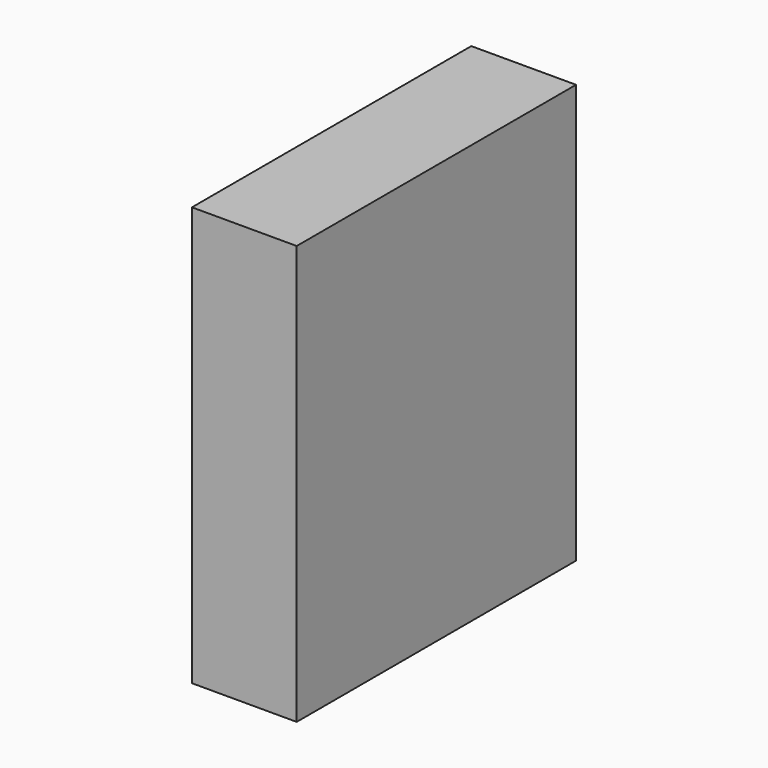
from build123d import *

# Parameters (mm, degrees)
F0_W         = 300
F0_H         = 1000
F1_DEPTH     = 1200
F2_T         = -25
F3_W         = 50
F3_H         = 1150
F4_DEPTH     = 275
F5_TEXT_SIZE = 40.509013666
F6_DEPTH     = 10


# Not quite as in the source:
# - a feature names something its author has since deleted; it is built from what else it names
# - Text() gives the source's letters only with a copy of the font that has no kerning and outlines rounded to 1/6400 em; it was checked with that copy


with BuildPart() as f1:
    # F0 (on Top) → F1 (new body)
    with BuildSketch(Plane.XY):
        Rectangle(F0_W, F0_H)
    extrude(amount=F1_DEPTH)

    # F2
    f2_openings = [f1.faces().sort_by_distance(p)[0] for p in [
        (-150, 0, 600),
    ]]
    offset(amount=F2_T, openings=f2_openings)

    # F3 (on face) → F4 (join)
    with BuildSketch(Plane(origin=(125, 0, 0), x_dir=(0, -1, 0), z_dir=(-1, 0, 0))):
        with Locations((190.852278471, 600)):
            Rectangle(F3_W, F3_H)
        with Locations((-180.2186727524, 600)):
            Rectangle(F3_W, F3_H)
    extrude(amount=F4_DEPTH)

    # F5 (on face) → F6 (join)
    with BuildSketch(Plane(origin=(0, 0, 0), x_dir=(1, 0, 0), z_dir=(0, 0, -1))):
        with Locations((-90.1935100555, 359.3434989452)):
            Text("David's", F5_TEXT_SIZE, font='Open Sans', text_align=(TextAlign.LEFT, TextAlign.BOTTOM))
        with Locations((-90.1935100555, 304.2512403594)):
            Text('Bookcase', F5_TEXT_SIZE, font='Open Sans', text_align=(TextAlign.LEFT, TextAlign.BOTTOM))
    extrude(amount=F6_DEPTH)


solid = f1.part
